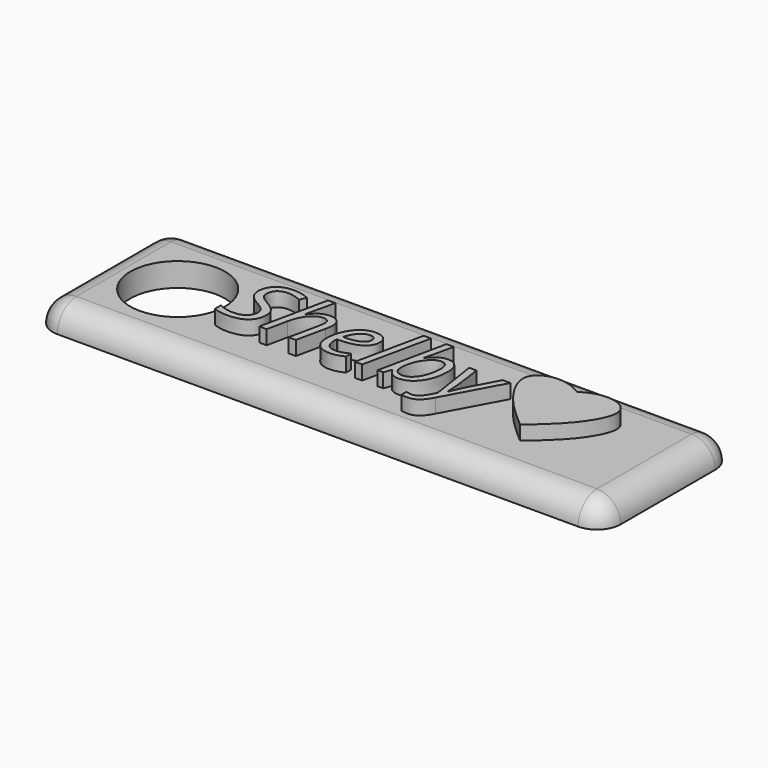
from build123d import *

# Parameters (mm, degrees)
F0_W         = 120
F0_H         = 35
F0_R         = 10
F1_DEPTH     = 5
F2_R         = 5
F3_R         = 5
F4_R         = 5
F5_R         = 5
F6_R         = 4.99999
F7_TEXT_SIZE = 18.88489286
F8_DEPTH     = 3
F10_DEPTH    = 3


# Not quite as in the source:
# - a fillet or chamfer is up to 0.001 mm smaller than in the source, because OpenCascade refuses the exact size
# - Text() gives the source's letters only with a copy of the font that has no kerning and outlines rounded to 1/6400 em; it was checked with that copy


with BuildPart() as f1:
    # F0 (on Top) → F1 (new body)
    with BuildSketch(Plane.XY):
        Rectangle(F0_W, F0_H)
        with Locations((-43.5899487349, 0)):
            Circle(F0_R, mode=Mode.SUBTRACT)
    extrude(amount=F1_DEPTH)

    # F2
    f2_edges = [f1.edges().sort_by_distance(p)[0] for p in [
        (-60, -17.5, 2.5),
    ]]
    fillet(f2_edges, radius=F2_R)

    # F3
    f3_edges = [f1.edges().sort_by_distance(p)[0] for p in [
        (-60, 17.5, 2.5),
    ]]
    fillet(f3_edges, radius=F3_R)

    # F4
    f4_edges = [f1.edges().sort_by_distance(p)[0] for p in [
        (60, 17.5, 2.5),
    ]]
    fillet(f4_edges, radius=F4_R)

    # F5
    f5_edges = [f1.edges().sort_by_distance(p)[0] for p in [
        (60, -17.5, 2.5),
    ]]
    fillet(f5_edges, radius=F5_R)

    # F6 (radius 5 in the source; OpenCascade refuses exactly that, so slightly less here)
    f6_edges = [f1.edges().sort_by_distance(p)[0] for p in [
        (-60, 0, 5),
    ]]
    fillet(f6_edges, radius=F6_R)

    # F7 (on face) → F8 (join)
    with BuildSketch(Plane.XY.offset(5)):
        with Locations((-31.1600724235, -6.5152877942)):
            Text('Shelby', F7_TEXT_SIZE, font='Open Sans', font_style=FontStyle.ITALIC, text_align=(TextAlign.LEFT, TextAlign.BOTTOM))
    extrude(amount=F8_DEPTH)

    # F9 (on face) → F10 (join)
    with BuildSketch(Plane.XY.offset(5)):
        with BuildLine():
            add(Edge.make_bspline(
                [(34.3683026731, 7.9903500155), (35.1779933178, 8.4702032401), (36.9788500169, 9.537458864), (41.6295039676, 9.9157102098), (45.2717485981, 6.9228531714), (42.7107468004, 1.2251611276), (38.7405570423, -3.2690770251), (35.8043483194, -5.7901355838), (34.3683026731, -7.0231389254)],
                knots=[0, 0, 0, 0, 0.1329428104, 0.2956820018, 0.444013085, 0.623375644, 0.8157999592, 1, 1, 1, 1], degree=3))
            add(Edge.make_bspline(
                [(34.3683026731, 7.9903500155), (33.5586120284, 8.4702032401), (31.7577553294, 9.537458864), (27.1071013786, 9.9157102098), (23.4648567481, 6.9228531714), (26.0258585458, 1.2251611276), (29.9960483039, -3.2690770251), (32.9322570268, -5.7901355838), (34.3683026731, -7.0231389254)],
                knots=[0, 0, 0, 0, 0.1329428104, 0.2956820018, 0.444013085, 0.623375644, 0.8157999592, 1, 1, 1, 1], degree=3))
        make_face()
    extrude(amount=F10_DEPTH)


solid = f1.part
